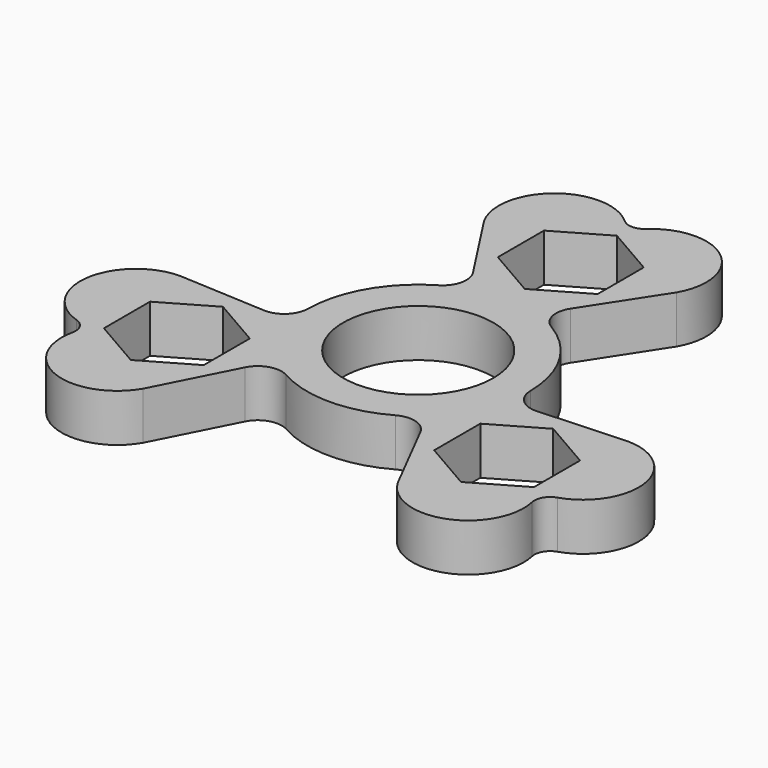
from build123d import *

# Parameters (mm, degrees)
F0_R     = 14
F0_R_2   = 9.45
F1_DEPTH = 6
F3_DEPTH = 6


# Not quite as in the source:
# - a feature names something its author has since deleted; it is built from what else it names


with BuildPart() as f1:
    # F0 (on Top) → F1 (new body)
    with BuildSketch(Plane.XY):
        Circle(F0_R)
        Circle(F0_R_2, mode=Mode.SUBTRACT)
    extrude(amount=F1_DEPTH)

    # F2 (on Top) → F3 (join)
    with BuildSketch(Plane.XY):
        with BuildLine():
            ThreePointArc((7.1208542294, 12.0537726478), (5.7261776623, 13.9509775601), (6.1307398604, 16.2706410345))
            Line((6.1307398604, 16.2706410345), (12.124355653, 25.5))
            ThreePointArc((12.124355653, 25.5), (10.4510884103, 34.4532067527), (1.3471506281, 34.1738301594))
            ThreePointArc((1.3471506281, 34.1738301594), (0, 33.6520673478), (-1.3471506281, 34.1738301594))
            ThreePointArc((-1.3471506281, 34.1738301594), (-10.4510884103, 34.4532067527), (-12.124355653, 25.5))
            Line((-12.124355653, 25.5), (-6.1307398604, 16.2706410345))
            ThreePointArc((-6.1307398604, 16.2706410345), (-5.7261776623, 13.9509775601), (-7.1208542294, 12.0537726478))
            ThreePointArc((-7.1208542294, 12.0537726478), (0, 14), (7.1208542294, 12.0537726478))
        make_face()
        Polygon((-6.2786841774, 27.625), (0, 31.25), (6.2786841774, 27.625), (6.2786841774, 20.375), (0, 16.75), (-6.2786841774, 20.375), align=None, mode=Mode.SUBTRACT)
        with BuildLine():
            ThreePointArc((17.1561584019, -2.8259440541), (14.9449898058, -2.016473458), (13.9993004391, 0.1399543354))
            ThreePointArc((13.9993004391, 0.1399543354), (13.9998251087, 0.0699780419), (14, 0))
            ThreePointArc((14, 0), (12.0892151717, -7.0605153163), (6.8784462097, -12.1937269832))
            ThreePointArc((6.8784462097, -12.1937269832), (9.2188121436, -11.9345041022), (11.0254185415, -13.4446969803))
            Line((11.0254185415, -13.4446969803), (16.02146997, -23.25))
            ThreePointArc((16.02146997, -23.25), (24.6118080845, -26.2775114368), (28.9218297486, -18.2535817464))
            ThreePointArc((28.9218297486, -18.2535817464), (29.1435452131, -16.8260336739), (30.2689803767, -15.920248413))
            ThreePointArc((30.2689803767, -15.920248413), (35.0628964948, -8.1756953159), (28.145825623, -2.25))
            Line((28.145825623, -2.25), (17.1561584019, -2.8259440541))
        make_face()
        Polygon((27.0632938683, -15.625), (20.7846096908, -19.25), (14.5059255134, -15.625), (14.5059255134, -8.375), (20.7846096908, -4.75), (27.0632938683, -8.375), align=None, mode=Mode.SUBTRACT)
        with BuildLine():
            ThreePointArc((-6.8784462097, -12.1937269832), (-12.124355653, -7), (-13.9993004391, 0.1399543354))
            ThreePointArc((-13.9993004391, 0.1399543354), (-14.9449898058, -2.016473458), (-17.1561584019, -2.8259440541))
            Line((-17.1561584019, -2.8259440541), (-28.145825623, -2.25))
            ThreePointArc((-28.145825623, -2.25), (-35.0628964948, -8.1756953159), (-30.2689803767, -15.920248413))
            ThreePointArc((-30.2689803767, -15.920248413), (-29.1435452131, -16.8260336739), (-28.9218297486, -18.2535817464))
            ThreePointArc((-28.9218297486, -18.2535817464), (-24.6118080845, -26.2775114368), (-16.02146997, -23.25))
            Line((-16.02146997, -23.25), (-11.0254185415, -13.4446969803))
            ThreePointArc((-11.0254185415, -13.4446969803), (-9.2188121436, -11.9345041022), (-6.8784462097, -12.1937269832))
        make_face()
        Polygon((-27.0632938683, -15.625), (-27.0632938683, -8.375), (-20.7846096908, -4.75), (-14.5059255134, -8.375), (-14.5059255134, -15.625), (-20.7846096908, -19.25), align=None, mode=Mode.SUBTRACT)
    extrude(amount=F3_DEPTH)


solid = f1.part
